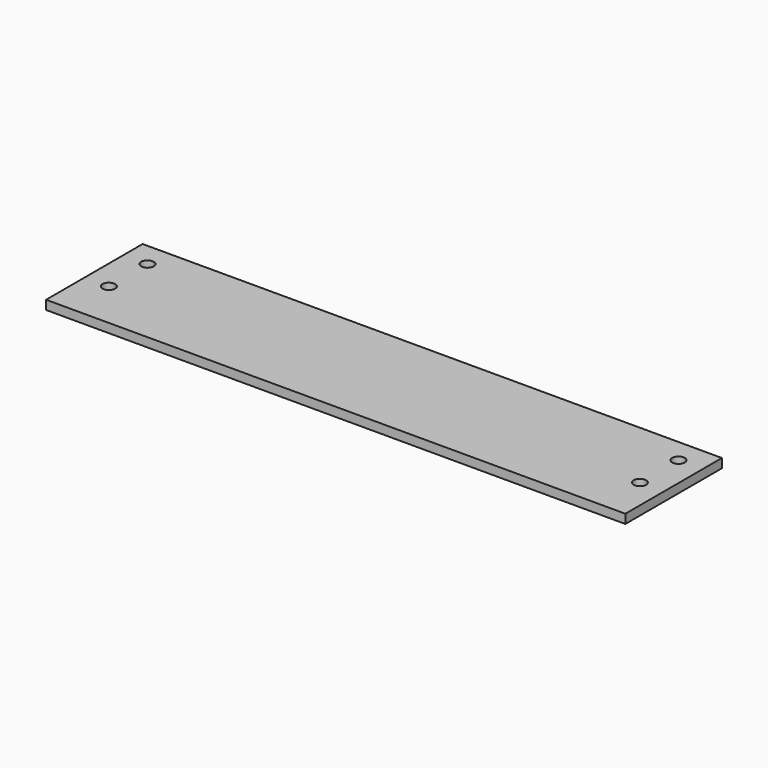
from build123d import *

# Parameters (mm, degrees)
F0_W     = 304.8
F0_H     = 63.5
F0_R     = 3.302
F1_DEPTH = 4.7625


# Not quite as in the source:
# - a length typed as a fraction of an inch, garbled in the dataset ("3 / 203.2 mm" for 3/8 in), is restored


with BuildPart() as f1:
    # F0 (on Top) → F1 (new body)
    with BuildSketch(Plane.XY):
        Rectangle(F0_W, F0_H)
        with Locations((-139.7, -6.35)):
            Circle(F0_R, mode=Mode.SUBTRACT)
        with Locations((139.7, -6.35)):
            Circle(F0_R, mode=Mode.SUBTRACT)
        with Locations((-139.7, 19.05)):
            Circle(F0_R, mode=Mode.SUBTRACT)
        with Locations((139.7, 19.05)):
            Circle(F0_R, mode=Mode.SUBTRACT)
    extrude(amount=F1_DEPTH)


solid = f1.part
